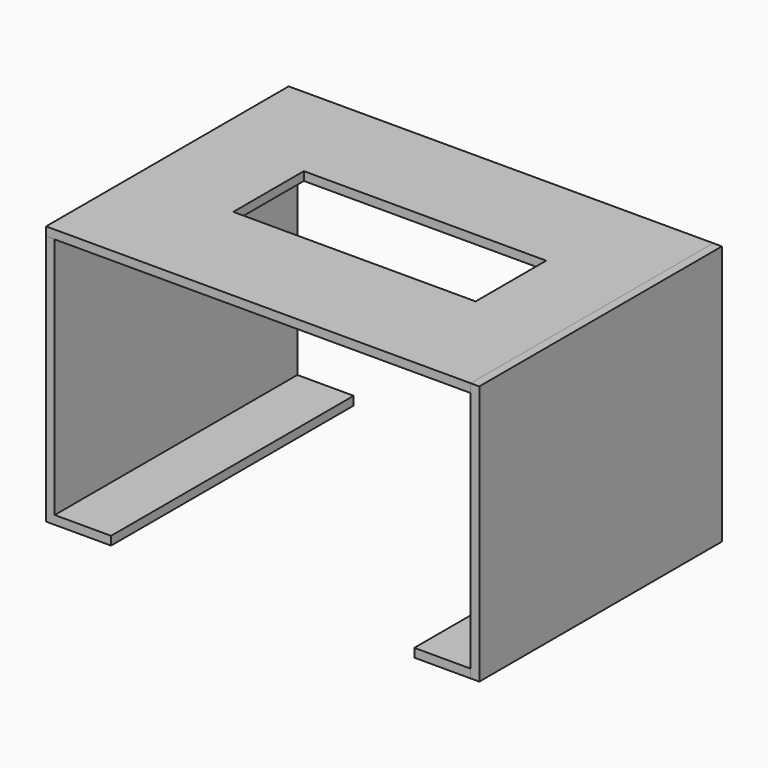
from build123d import *

# Parameters (mm, degrees)
F1_E0_W  = 15
F1_E0_H  = 70
F2_DEPTH = 2
F1_E4_W  = 15
F1_E4_H  = 70
F1_E1_W  = 60
F1_E1_H  = 70
F3_DEPTH = 2
F1_E2_W  = 100
F1_E2_H  = 70
F4_DEPTH = 2
F1_E3_W  = 60
F1_E3_H  = 70
F5_DEPTH = 2
F6_W     = 55.9396576136
F6_H     = 20.3663799912
F7_DEPTH = 30.9466302677


with BuildPart() as f2:
    # F1_E0 (on explicit) → F2 (new body)
    with BuildSketch(Plane(origin=(-37.1421206879, 35, -29.0543697323), x_dir=(-1, 0, 0), z_dir=(0, 0, 1))):
        with Locations((7.5, 35)):
            Rectangle(F1_E0_W, F1_E0_H)
    extrude(amount=F2_DEPTH)

    # F1_E1 (on explicit) → F3 (join)
    with BuildSketch(Plane(origin=(-52.1421206879, 35, -29.0543697323), x_dir=(0, 0, 1), z_dir=(1, 0, 0))):
        with Locations((30, 35)):
            Rectangle(F1_E1_W, F1_E1_H)
    extrude(amount=F3_DEPTH)


with BuildPart() as f2b:
    # F1_E4 (on explicit) → F2, piece 2 (new body)
    with BuildSketch(Plane(origin=(47.8578793121, 35, -29.0543697323), x_dir=(-1, 0, 0), z_dir=(0, 0, 1))):
        with Locations((7.5, 35)):
            Rectangle(F1_E4_W, F1_E4_H)
    extrude(amount=F2_DEPTH)


with BuildPart() as f4:
    # F1_E2 (on explicit) → F4 (new body)
    with BuildSketch(Plane(origin=(-52.1421206879, 35, 30.9456302677), x_dir=(1, 0, 0), z_dir=(0, 0, -1))):
        with Locations((50, 35)):
            Rectangle(F1_E2_W, F1_E2_H)
    extrude(amount=F4_DEPTH)

    # F6 (on Top) → F7 (cut, through all)
    with BuildSketch(Plane.XY):
        with Locations((-1.357759349, 0.6788792089)):
            Rectangle(F6_W, F6_H)
    extrude(amount=F7_DEPTH, mode=Mode.SUBTRACT)


with BuildPart() as f5:
    # F1_E3 (on explicit) → F5 (new body)
    with BuildSketch(Plane(origin=(47.8578793121, 35, 30.9456302677), x_dir=(0, 0, -1), z_dir=(-1, 0, 0))):
        with Locations((30, 35)):
            Rectangle(F1_E3_W, F1_E3_H)
    extrude(amount=F5_DEPTH)


solid = Compound([f2.part, f2b.part, f4.part, f5.part])
